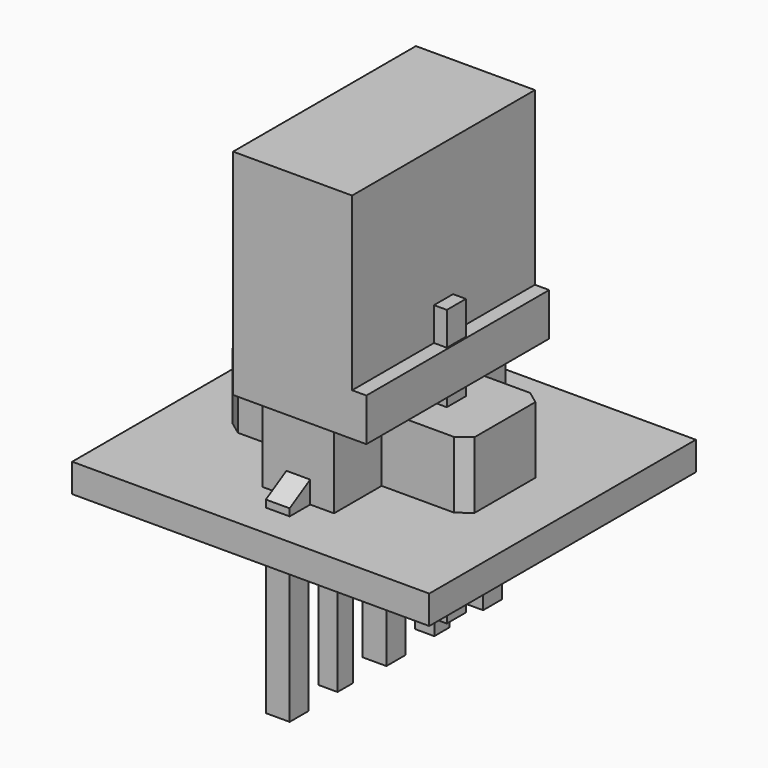
from build123d import *

# Parameters (mm, degrees)
F2_DEPTH       = 2.4
F3_W           = 0.5
F3_H           = 5.4
F4_DEPTH       = 0.25
F5_W           = 4.5
F5_H           = 5.7
F6_DEPTH       = 0.75
F9_W           = 0.4
F9_H           = 3.2
F10_DEPTH      = 0.2
F11_W          = 0.5
F11_H          = 0.5
F12_DEPTH      = 2
F13_W          = 0.5
F13_H          = 0.5
F14_DEPTH      = 1.8
F14_DEPTH_BACK = 4
F15_W          = 7.5
F15_H          = 7
F16_DEPTH      = 0.6


with BuildPart() as f2:
    # F1 (on Front) → F2 (new body, symmetric)
    with BuildSketch(Plane.XZ):
        Polygon((1.25, 6.7), (-1.25, 6.7), (-1.25, 2.2), (1.55, 2.2), (1.55, 3.1), (1.25, 3.1), align=None)
    extrude(amount=F2_DEPTH, both=True)

    # F3 (on Right) → F4 (join, symmetric)
    with BuildSketch(Plane.YZ):
        with Locations((0, -0.5)):
            Rectangle(F3_W, F3_H)
        Polygon((1.75, 2.2), (1.25, 2.2), (1.25, 0), (2.29, 0), (2.29, -3.2), (2.79, -3.2), (2.79, 0.5), (1.75, 0.5), align=None)
        Polygon((-1.25, 2.2), (-1.75, 2.2), (-1.75, 1.35044428), (-2.79, 0.75), (-2.79, -3.2), (-2.29, -3.2), (-2.29, 0), (-1.25, 0), align=None)
    extrude(amount=F4_DEPTH, both=True)


with BuildPart() as f6:
    # F5 (on Right) → F6 (new body, symmetric)
    with BuildSketch(Plane.YZ):
        with Locations((0, 2.85)):
            Rectangle(F5_W, F5_H)
    extrude(amount=F6_DEPTH, both=True)

    # F7 (on face) → F8 (revolve)
    with BuildSketch(Plane(origin=(-0.75, 0, 0), x_dir=(0, -1, 0), z_dir=(-1, 0, 0))):
        with BuildLine():
            Line((0, 3.75), (0, 5.25))
            ThreePointArc((0, 5.25), (-0.75, 4.5), (0, 3.75))
        make_face()
    revolve(axis=Axis((-0.75, 0, 4.5), (0, 0, -1)))

    # F9 (on Right) → F10 (join, symmetric)
    with BuildSketch(Plane.YZ):
        with Locations((1.27, -1.6)):
            Rectangle(F9_W, F9_H)
        with Locations((-1.27, -1.6)):
            Rectangle(F9_W, F9_H)
    extrude(amount=F10_DEPTH, both=True)


with BuildPart() as f12:
    # F11 (on Top) → F12 (new body)
    with BuildSketch(Plane.XY):
        Polygon((0.27, 1), (0, 0.8), (0, -0.8), (0.27, -1), (2.27, -1), (2.54, -0.8), (2.54, 0.8), (2.27, 1), align=None)
        with Locations((1.27, 0)):
            Rectangle(F11_W, F11_H, mode=Mode.SUBTRACT)
        Polygon((0, -0.8), (0, 0.8), (-0.27, 1), (-2.27, 1), (-2.54, 0.8), (-2.54, -0.8), (-2.27, -1), (-0.27, -1), align=None)
        with Locations((-1.27, 0)):
            Rectangle(F11_W, F11_H, mode=Mode.SUBTRACT)
    extrude(amount=F12_DEPTH)

    # F13 (on face) → F14 (join, two sides)
    with BuildSketch(Plane.XY.offset(2)) as f14_sk:
        with Locations((1.27, 0)):
            Rectangle(F13_W, F13_H)
        with Locations((-1.27, 0)):
            Rectangle(F13_W, F13_H)
    extrude(amount=F14_DEPTH)
    extrude(f14_sk.sketch, amount=-F14_DEPTH_BACK)


with BuildPart() as f16:
    # F15 (on Top) → F16 (new body)
    with BuildSketch(Plane.XY):
        Rectangle(F15_W, F15_H)
    extrude(amount=F16_DEPTH)


solid = Compound([f2.part, f6.part, f12.part, f16.part])
